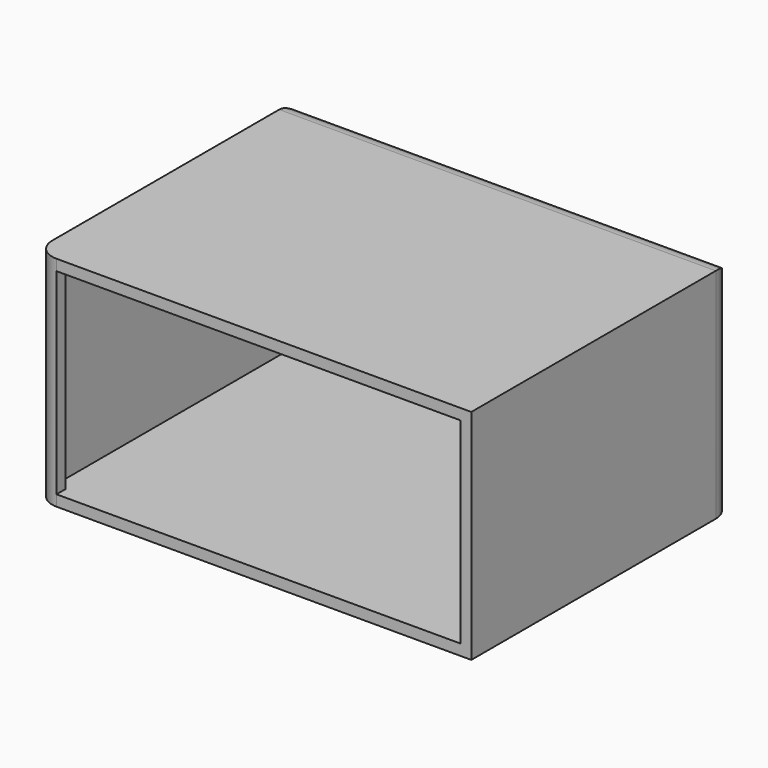
from build123d import *

# Parameters (mm, degrees)
F0_W     = 101.6
F0_H     = 50.8
F1_DEPTH = 76.2
F2_R     = 5.08
F3_T     = -2.54


# Not quite as in the source:
# - a shell that OpenCascade refuses in one call is made with other operations: the cavity is built on its own and cut out


with BuildPart() as f1:
    # F0 (on Front) → F1 (new body)
    with BuildSketch(Plane.XZ):
        with Locations((11.4285616755, 25.4)):
            Rectangle(F0_W, F0_H)
    extrude(amount=F1_DEPTH)

    # F2
    f2_edges = [f1.edges().sort_by_distance(p)[0] for p in [
        (-39.371438, -76.2, 25.4),
        (-39.371438, 0, 25.4),
        (11.428562, 0, 50.8),
        (62.228562, 0, 25.4),
    ]]
    fillet(f2_edges, radius=F2_R)

    # F3: a shell. OpenCascade refuses it in one call, so the cavity is built on its own and cut out:
    # the body offset inwards by the wall thickness, plus a prism from it out through each open face.
    f3_core = offset(f1.part, amount=F3_T, mode=Mode.PRIVATE)
    f3_exits = [f3_core.faces().sort_by_distance(p)[0] for p in [
        (12.698562, -73.66, 25.4),
    ]]
    add(f3_core, mode=Mode.SUBTRACT)
    extrude(f3_exits, amount=-F3_T, mode=Mode.SUBTRACT)


solid = f1.part
